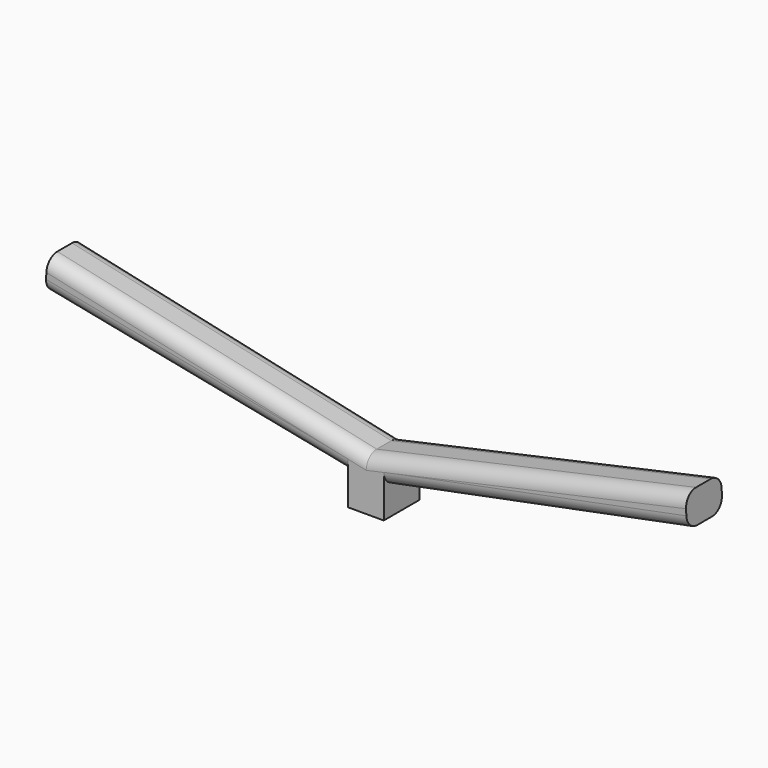
from build123d import *

# Parameters (mm, degrees)
F1_DEPTH     = 17.272
F2_T4_DEPTH  = 145.1755034497
F2_T9_DEPTH  = 145.1755034497
F2_T14_DEPTH = 145.451805042
F2_T19_DEPTH = 145.451805042
F2_T24_DEPTH = 152.4
F2_T29_DEPTH = 152.4
F2_T34_DEPTH = 152.4
F2_T39_DEPTH = 152.4
F2_T45_DEPTH = 152.4
F2_T49_DEPTH = 152.4
F2_T56_DEPTH = 152.4
F2_T60_DEPTH = 152.4


# Not quite as in the source:
# - a fillet or chamfer that OpenCascade refuses, or shapes differently, is made with other operations: its cross-section is extruded or revolved along the edge and cut away or added


with BuildPart() as f1:
    # F0 (on Front) → F1 (new body)
    with BuildSketch(Plane.XZ):
        Polygon((-58.1587258462, 60.3411067049), (-182.2034080142, 87.5792568958), (-182.731828862, 74.8902549096), (-65.2451664209, 51.5867063582), (-65.2451664209, 57.4221499264), (-51.3433068991, 57.4221499264), (-51.3433068991, 51.5329490591), (66.4143771697, 74.8902549096), (65.8859563219, 87.5792568958), align=None)
        Polygon((-65.2451664209, 57.4221499264), (-65.2451664209, 51.5867063582), (-58.1587258462, 50.1811067049), (-51.3433068991, 51.5329490591), (-51.3433068991, 57.4221499264), align=None)
        Polygon((-58.1587258462, 50.1811067049), (-65.2451664209, 51.5867063582), (-65.2451664209, 40.1959307492), (-51.3433068991, 40.1959307492), (-51.3433068991, 51.5329490591), align=None)
    extrude(amount=-F1_DEPTH)

    # F2: fillet of radius 5.08 on 8 edges, made by hand


with BuildPart() as f2_tool2:
    # F2_s3 → F2_t4 (new body)
    with BuildSketch(Plane(origin=(-202.5642945881, 0, 40.1787468945), x_dir=(0, 1, 0), z_dir=(0.9808905749, 0, -0.1945602221))):
        with BuildLine():
            ThreePointArc((12.192, 37.9067999896), (15.7841024484, 39.3946975412), (17.272, 42.9867999896))
            Line((17.272, 42.9867999896), (17.272, 37.9067999896))
            Line((17.272, 37.9067999896), (12.192, 37.9067999896))
        make_face()
    extrude(amount=F2_T4_DEPTH)

    split(bisect_by=Plane.YZ.offset(-65.2451664209), keep=Keep.BOTTOM)


with BuildPart() as f1_1:
    add(f1.part)

    # F2_t1: cut F2_tool2
    add(f2_tool2.part, mode=Mode.SUBTRACT)


with BuildPart() as f2_tool7:
    # F2_s8 → F2_t9 (new body)
    with BuildSketch(Plane(origin=(-202.5642945881, 0, 40.1787468945), x_dir=(0, 1, 0), z_dir=(0.9808905749, 0, -0.1945602221))):
        with BuildLine():
            ThreePointArc((5.08, 37.9067999896), (1.4878975516, 39.3946975412), (0, 42.9867999896))
            Line((0, 42.9867999896), (0, 37.9067999896))
            Line((0, 37.9067999896), (5.08, 37.9067999896))
        make_face()
    extrude(amount=F2_T9_DEPTH)

    split(bisect_by=Plane.YZ.offset(-65.2451664209), keep=Keep.BOTTOM)


with BuildPart() as f1_2:
    add(f1_1.part)

    # F2_t6: cut F2_tool7
    add(f2_tool7.part, mode=Mode.SUBTRACT)


with BuildPart() as f2_tool12:
    # F2_s13 → F2_t14 (new body)
    with BuildSketch(Plane(origin=(-52.0224181794, 0, -10.3186772236), x_dir=(0, 1, 0), z_dir=(0.9808905749, 0, 0.1945602221))):
        with BuildLine():
            ThreePointArc((12.192, 60.5375492231), (15.7841024484, 62.0254467746), (17.272, 65.6175492231))
            Line((17.272, 65.6175492231), (17.272, 60.5375492231))
            Line((17.272, 60.5375492231), (12.192, 60.5375492231))
        make_face()
    extrude(amount=F2_T14_DEPTH)

    split(bisect_by=Plane.YZ.offset(-51.3433068991), keep=Keep.TOP)


with BuildPart() as f1_3:
    add(f1_2.part)

    # F2_t11: cut F2_tool12
    add(f2_tool12.part, mode=Mode.SUBTRACT)


with BuildPart() as f2_tool17:
    # F2_s18 → F2_t19 (new body)
    with BuildSketch(Plane(origin=(-52.0224181794, 0, -10.3186772236), x_dir=(0, 1, 0), z_dir=(0.9808905749, 0, 0.1945602221))):
        with BuildLine():
            ThreePointArc((5.08, 60.5375492231), (1.4878975516, 62.0254467746), (0, 65.6175492231))
            Line((0, 65.6175492231), (0, 60.5375492231))
            Line((0, 60.5375492231), (5.08, 60.5375492231))
        make_face()
    extrude(amount=F2_T19_DEPTH)

    split(bisect_by=Plane.YZ.offset(-51.3433068991), keep=Keep.TOP)


with BuildPart() as f1_4:
    add(f1_3.part)

    # F2_t16: cut F2_tool17
    add(f2_tool17.part, mode=Mode.SUBTRACT)


with BuildPart() as f2_tool22:
    # F2_s23 → F2_t24 (new body)
    with BuildSketch(Plane(origin=(-55.7194406669, 0, 12.2350629379), x_dir=(0, 1, 0), z_dir=(-0.9767297809, 0, 0.2144736236))):
        with BuildLine():
            ThreePointArc((12.192, -46.4634432549), (15.7841024484, -44.9755457034), (17.272, -41.3834432549))
            Line((17.272, -41.3834432549), (17.272, -46.4634432549))
            Line((17.272, -46.4634432549), (12.192, -46.4634432549))
        make_face()
    extrude(amount=F2_T24_DEPTH)

    split(bisect_by=Plane(origin=(-15.3156619604, 0, 69.7487313476), x_dir=(0, 1, 0), z_dir=(-0.2144736236, 0, 0.9767297809)), keep=Keep.TOP)


with BuildPart() as f1_5:
    add(f1_4.part)

    # F2_t21: cut F2_tool22
    add(f2_tool22.part, mode=Mode.SUBTRACT)


with BuildPart() as f2_tool27:
    # F2_s28 → F2_t29 (new body)
    with BuildSketch(Plane(origin=(-55.7194406669, 0, 12.2350629379), x_dir=(0, 1, 0), z_dir=(-0.9767297809, 0, 0.2144736236))):
        with BuildLine():
            ThreePointArc((5.08, -46.4634432549), (1.4878975516, -44.9755457034), (0, -41.3834432549))
            Line((0, -41.3834432549), (0, -46.4634432549))
            Line((0, -46.4634432549), (5.08, -46.4634432549))
        make_face()
    extrude(amount=F2_T29_DEPTH)

    split(bisect_by=Plane(origin=(-15.3156619604, 0, 69.7487313476), x_dir=(0, 1, 0), z_dir=(-0.2144736236, 0, 0.9767297809)), keep=Keep.TOP)


with BuildPart() as f1_6:
    add(f1_5.part)

    # F2_t26: cut F2_tool27
    add(f2_tool27.part, mode=Mode.SUBTRACT)


with BuildPart() as f2_tool32:
    # F2_s33 → F2_t34 (new body)
    with BuildSketch(Plane(origin=(93.6060864991, 0, 20.5543405673), x_dir=(0, 1, 0), z_dir=(-0.9767297809, 0, -0.2144736236))):
        with BuildLine():
            ThreePointArc((5.08, -71.4104686015), (1.4878975516, -69.92257105), (0, -66.3304686015))
            Line((0, -66.3304686015), (0, -71.4104686015))
            Line((0, -71.4104686015), (5.08, -71.4104686015))
        make_face()
    extrude(amount=F2_T34_DEPTH)

    split(bisect_by=Plane(origin=(9.9651830375, 0, 45.382228748), x_dir=(0, 1, 0), z_dir=(0.2144736236, 0, 0.9767297809)), keep=Keep.TOP)


with BuildPart() as f1_7:
    add(f1_6.part)

    # F2_t31: cut F2_tool32
    add(f2_tool32.part, mode=Mode.SUBTRACT)


with BuildPart() as f2_tool37:
    # F2_s38 → F2_t39 (new body)
    with BuildSketch(Plane(origin=(93.6060864991, 0, 20.5543405673), x_dir=(0, 1, 0), z_dir=(-0.9767297809, 0, -0.2144736236))):
        with BuildLine():
            ThreePointArc((12.192, -71.4104686015), (15.7841024484, -69.92257105), (17.272, -66.3304686015))
            Line((17.272, -66.3304686015), (17.272, -71.4104686015))
            Line((17.272, -71.4104686015), (12.192, -71.4104686015))
        make_face()
    extrude(amount=F2_T39_DEPTH)

    split(bisect_by=Plane(origin=(9.9651830375, 0, 45.382228748), x_dir=(0, 1, 0), z_dir=(0.2144736236, 0, 0.9767297809)), keep=Keep.TOP)


with BuildPart() as f1_8:
    add(f1_7.part)

    # F2_t36: cut F2_tool37
    add(f2_tool37.part, mode=Mode.SUBTRACT)


with BuildPart() as f2_tool43:
    # F2_s44 → F2_t45 (new body)
    with BuildSketch(Plane(origin=(93.6060864991, 0, 20.5543405673), x_dir=(0, 1, 0), z_dir=(-0.9767297809, 0, -0.2144736236))):
        with BuildLine():
            ThreePointArc((12.192, -71.4104686015), (15.7841024484, -69.92257105), (17.272, -66.3304686015))
            Line((17.272, -66.3304686015), (17.272, -71.4104686015))
            Line((17.272, -71.4104686015), (12.192, -71.4104686015))
        make_face()
    extrude(amount=F2_T45_DEPTH)

    split(bisect_by=Plane(origin=(9.9651830375, 0, 45.382228748), x_dir=(0, 1, 0), z_dir=(-0.2144736236, 0, -0.9767297809)), keep=Keep.TOP)


with BuildPart() as f2_tool47:
    # F2_s48 → F2_t49 (new body)
    with BuildSketch(Plane(origin=(-55.7194406669, 0, 12.2350629379), x_dir=(0, 1, 0), z_dir=(-0.9767297809, 0, 0.2144736236))):
        with BuildLine():
            ThreePointArc((12.192, -46.4634432549), (15.7841024484, -44.9755457034), (17.272, -41.3834432549))
            Line((17.272, -41.3834432549), (17.272, -46.4634432549))
            Line((17.272, -46.4634432549), (12.192, -46.4634432549))
        make_face()
    extrude(amount=F2_T49_DEPTH)

    split(bisect_by=Plane(origin=(-15.3156619604, 0, 69.7487313476), x_dir=(0, 1, 0), z_dir=(0.2144736236, 0, -0.9767297809)), keep=Keep.TOP)


with BuildPart() as f2_tool43_1:
    add(f2_tool43.part)

    # F2_t51: intersect F2_tool47
    add(f2_tool47.part, mode=Mode.INTERSECT)


with BuildPart() as f1_9:
    add(f1_8.part)

    # F2_t41: cut F2_tool43
    add(f2_tool43_1.part, mode=Mode.SUBTRACT)


with BuildPart() as f2_tool54:
    # F2_s55 → F2_t56 (new body)
    with BuildSketch(Plane(origin=(93.6060864991, 0, 20.5543405673), x_dir=(0, 1, 0), z_dir=(-0.9767297809, 0, -0.2144736236))):
        with BuildLine():
            ThreePointArc((5.08, -71.4104686015), (1.4878975516, -69.92257105), (0, -66.3304686015))
            Line((0, -66.3304686015), (0, -71.4104686015))
            Line((0, -71.4104686015), (5.08, -71.4104686015))
        make_face()
    extrude(amount=F2_T56_DEPTH)

    split(bisect_by=Plane(origin=(9.9651830375, 0, 45.382228748), x_dir=(0, 1, 0), z_dir=(-0.2144736236, 0, -0.9767297809)), keep=Keep.TOP)


with BuildPart() as f2_tool58:
    # F2_s59 → F2_t60 (new body)
    with BuildSketch(Plane(origin=(-55.7194406669, 0, 12.2350629379), x_dir=(0, 1, 0), z_dir=(-0.9767297809, 0, 0.2144736236))):
        with BuildLine():
            ThreePointArc((5.08, -46.4634432549), (1.4878975516, -44.9755457034), (0, -41.3834432549))
            Line((0, -41.3834432549), (0, -46.4634432549))
            Line((0, -46.4634432549), (5.08, -46.4634432549))
        make_face()
    extrude(amount=F2_T60_DEPTH)

    split(bisect_by=Plane(origin=(-15.3156619604, 0, 69.7487313476), x_dir=(0, 1, 0), z_dir=(0.2144736236, 0, -0.9767297809)), keep=Keep.TOP)


with BuildPart() as f2_tool54_1:
    add(f2_tool54.part)

    # F2_t62: intersect F2_tool58
    add(f2_tool58.part, mode=Mode.INTERSECT)


with BuildPart() as f1_10:
    add(f1_9.part)

    # F2_t52: cut F2_tool54
    add(f2_tool54_1.part, mode=Mode.SUBTRACT)


solid = f1_10.part
